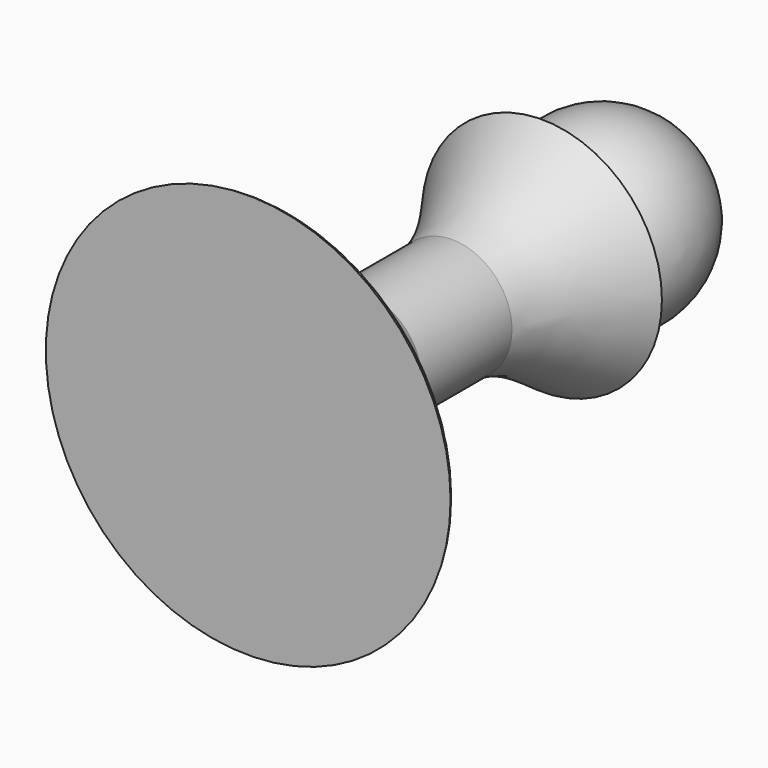
from build123d import *


with BuildPart() as f1:
    # F0 (on Top) → F1 (revolve)
    with BuildSketch(Plane.XY):
        with BuildLine():
            Line((40.64, 54.7711955523), (19.05, 54.7711955523))
            ThreePointArc((19.05, 54.7711955523), (30.1206947131, 90.2114271234), (0, 111.9211955523))
            Line((0, 111.9211955523), (0, -69.6888044477))
            Line((0, -69.6888044477), (68.58, -69.6888044477))
            add(Edge.make_bspline(
                [(60.96, -64.6088044477), (63.6417855309, -66.0841173211), (66.1108927654, -67.8864608844), (68.58, -69.6888044477)],
                knots=[0.8150158321, 0.8150158321, 0.8150158321, 0.8150158321, 1, 1, 1, 1], degree=3))
            Line((60.96, -64.6088044477), (50.8, -64.6088044477))
            Line((50.8, -64.6088044477), (50.8, -59.5288044477))
            add(Edge.make_bspline(
                [(20.32, -21.4288044477), (23.9114469199, -29.790276514), (30.8183636705, -45.8707011348), (45.2337782312, -56.4078117468), (50.8, -59.5288044477)],
                knots=[0, 0, 0, 0, 0.3166654052, 0.6089973318, 0.6089973318, 0.6089973318, 0.6089973318], degree=3))
            Line((20.32, -21.4288044477), (20.32, -10.7584101574))
            Line((20.32, -10.7584101574), (20.32, -10.1280333474))
            add(Edge.make_bspline(
                [(20.32, 16.6711955523), (18.2177086424, 5.9343622337), (20.2250450762, -5.4339231678), (20.32, -10.1280333474)],
                knots=[0.3403990237, 0.3403990237, 0.3403990237, 0.3403990237, 0.6085677542, 0.6085677542, 0.6085677542, 0.6085677542], degree=3))
            add(Edge.make_bspline(
                [(40.64, 54.7711955523), (32.2786703904, 42.9112967892), (22.9885360543, 30.2999567207), (20.32, 16.6711955523)],
                knots=[0, 0, 0, 0, 0.3403990237, 0.3403990237, 0.3403990237, 0.3403990237], degree=3))
        make_face()
        with BuildLine():
            Line((20.32, -10.1280333474), (20.32, 16.6711955523))
            add(Edge.make_bspline(
                [(20.32, 16.6711955523), (18.2177086424, 5.9343622337), (20.2250450762, -5.4339231678), (20.32, -10.1280333474)],
                knots=[0.3403990237, 0.3403990237, 0.3403990237, 0.3403990237, 0.6085677542, 0.6085677542, 0.6085677542, 0.6085677542], degree=3))
        make_face()
        with BuildLine():
            add(Edge.make_bspline(
                [(60.96, -64.6088044477), (63.6417855309, -66.0841173211), (66.1108927654, -67.8864608844), (68.58, -69.6888044477)],
                knots=[0.8150158321, 0.8150158321, 0.8150158321, 0.8150158321, 1, 1, 1, 1], degree=3))
            add(Edge.make_bspline(
                [(60.96, -64.6088044477), (64.9565607309, -64.943768084), (67.9345280908, -68.1189996069), (68.58, -69.6888044477)],
                knots=[0, 0, 0, 0, 0.7151272569, 0.7151272569, 0.7151272569, 0.7151272569], degree=3))
        make_face()
    revolve(axis=Axis((0, 21.1161955523, 0), (0, -1, 0)))


solid = f1.part
